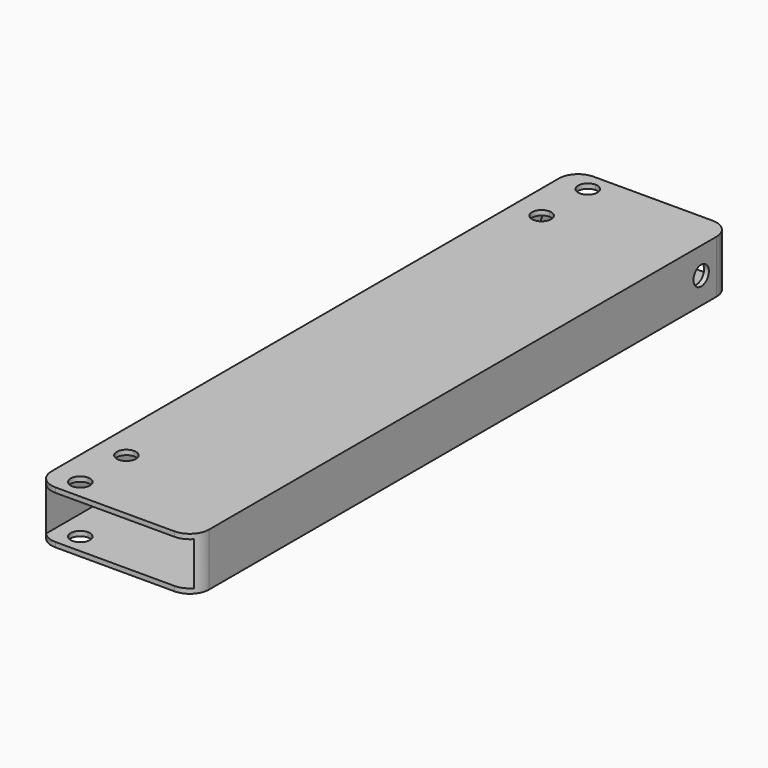
from build123d import *

# Parameters (mm, degrees)
F0_W        = 82
F0_H        = 27.5
F0_W_2      = 77
F0_H_2      = 22.5
F1_DEPTH    = 350
F3_DEPTH    = 53
F4_T1_DEPTH = 77.5
F5_R        = 5
F6_DEPTH    = 80.5


# Not quite as in the source:
# - a fillet or chamfer that OpenCascade refuses, or shapes differently, is made with other operations: its cross-section is extruded or revolved along the edge and cut away or added
# - a feature names something its author has since deleted; it is built from what else it names


with BuildPart() as f1:
    # F0 (on Front) → F1 (new body)
    with BuildSketch(Plane.XZ):
        with Locations((-33.9858543277, 13.75)):
            Rectangle(F0_W, F0_H)
        with Locations((-33.9858543277, 13.75)):
            Rectangle(F0_W_2, F0_H_2, mode=Mode.SUBTRACT)
    extrude(amount=F1_DEPTH)

    # F2 (on Top) → F3 (cut)
    with BuildSketch(Plane.XY):
        with BuildLine():
            Line((-59.9858543277, -340), (-59.9858543277, -335))
            ThreePointArc((-59.9858543277, -335), (-64.9858543277, -340), (-59.9858543277, -345))
            Line((-59.9858543277, -345), (-59.9858543277, -340))
        make_face()
        with BuildLine():
            ThreePointArc((-54.9858543277, -340), (-56.4503204217, -336.4644660941), (-59.9858543277, -335))
            Line((-59.9858543277, -335), (-59.9858543277, -340))
            Line((-59.9858543277, -340), (-59.9858543277, -345))
            ThreePointArc((-59.9858543277, -345), (-56.4503204217, -343.5355339059), (-54.9858543277, -340))
        make_face()
        with BuildLine():
            Line((-59.9858543277, -45), (-59.9858543277, -35))
            ThreePointArc((-59.9858543277, -35), (-64.9858543277, -40), (-59.9858543277, -45))
        make_face()
        with BuildLine():
            ThreePointArc((-54.9858543277, -40), (-56.4503204217, -36.4644660941), (-59.9858543277, -35))
            Line((-59.9858543277, -35), (-59.9858543277, -45))
            ThreePointArc((-59.9858543277, -45), (-56.4503204217, -43.5355339059), (-54.9858543277, -40))
        make_face()
        with BuildLine():
            Line((-59.9858543277, -15), (-59.9858543277, -5))
            ThreePointArc((-59.9858543277, -5), (-64.9858543277, -10), (-59.9858543277, -15))
        make_face()
        with BuildLine():
            ThreePointArc((-59.9858543277, -15), (-56.4503204217, -13.5355339059), (-54.9858543277, -10))
            ThreePointArc((-54.9858543277, -10), (-56.4503204217, -6.4644660941), (-59.9858543277, -5))
            Line((-59.9858543277, -5), (-59.9858543277, -15))
        make_face()
        with BuildLine():
            Line((-59.9858543277, -315), (-59.9858543277, -305))
            ThreePointArc((-59.9858543277, -305), (-64.9858543277, -310), (-59.9858543277, -315))
        make_face()
        with BuildLine():
            ThreePointArc((-54.9858543277, -310), (-56.4503204217, -306.4644660941), (-59.9858543277, -305))
            Line((-59.9858543277, -305), (-59.9858543277, -315))
            ThreePointArc((-59.9858543277, -315), (-56.4503204217, -313.5355339059), (-54.9858543277, -310))
        make_face()
    extrude(amount=F3_DEPTH, mode=Mode.SUBTRACT)

    # F4: fillet of radius 10 on 4 edges, made by hand

    # F4_s2 → F4_t1 (cut)
    with BuildSketch(Plane.XY.offset(-25)):
        with BuildLine():
            ThreePointArc((-64.9858543277, 0), (-72.0569221395, -2.9289321881), (-74.9858543277, -10))
            Line((-74.9858543277, -10), (-74.9858543277, 0))
            Line((-74.9858543277, 0), (-64.9858543277, 0))
        make_face()
        with BuildLine():
            ThreePointArc((-64.9858543277, -350), (-72.0569221395, -347.0710678119), (-74.9858543277, -340))
            Line((-74.9858543277, -340), (-74.9858543277, -350))
            Line((-74.9858543277, -350), (-64.9858543277, -350))
        make_face()
        with BuildLine():
            ThreePointArc((7.0141456723, -10), (4.0852134842, -2.9289321881), (-2.9858543277, 0))
            Line((-2.9858543277, 0), (7.0141456723, 0))
            Line((7.0141456723, 0), (7.0141456723, -10))
        make_face()
        with BuildLine():
            ThreePointArc((7.0141456723, -340), (4.0852134842, -347.0710678119), (-2.9858543277, -350))
            Line((-2.9858543277, -350), (7.0141456723, -350))
            Line((7.0141456723, -350), (7.0141456723, -340))
        make_face()
    extrude(amount=F4_T1_DEPTH, mode=Mode.SUBTRACT)

    # F5 (on face) → F6 (cut)
    with BuildSketch(Plane.YZ.offset(7.0141456723)):
        with Locations((-20, 13.75)):
            Circle(F5_R)
    extrude(amount=-F6_DEPTH, mode=Mode.SUBTRACT)


solid = f1.part
